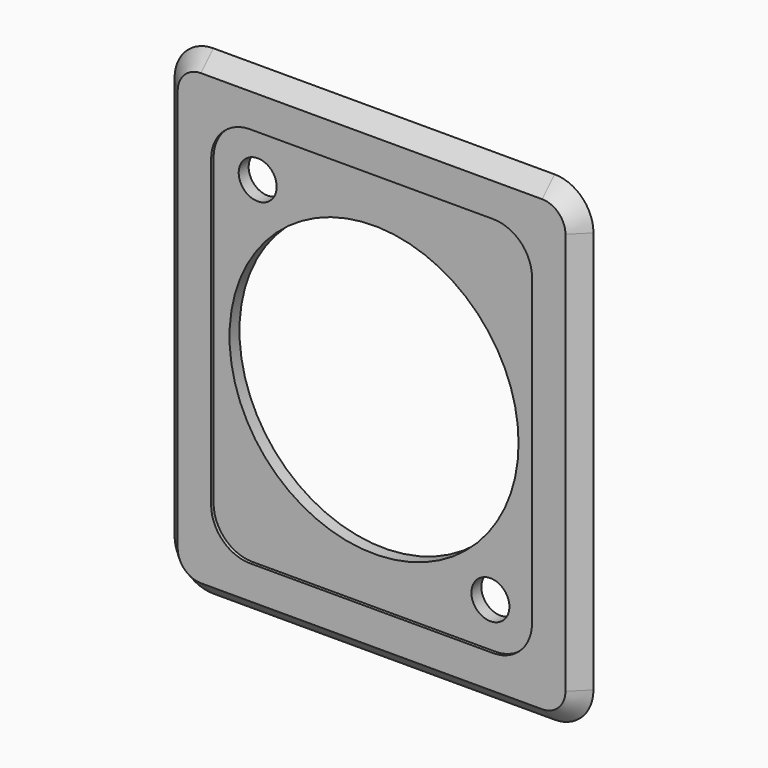
from build123d import *

# Parameters (mm, degrees)
F0_R     = 1.55
F0_R_2   = 11.8
F1_DEPTH = 1.27
F3_DEPTH = 0.254
F4_SIZE  = 1.26999


# Not quite as in the source:
# - a fillet or chamfer is up to 0.001 mm smaller than in the source, because OpenCascade refuses the exact size


with BuildPart() as f1:
    # F0 (on Front) → F1 (new body)
    with BuildSketch(Plane.XZ):
        with BuildLine():
            ThreePointArc((0, 3.175), (0.9299359697, 0.9299359697), (3.175, 0))
            Line((3.175, 0), (31.025, 0))
            ThreePointArc((31.025, 0), (33.2700640303, 0.9299359697), (34.2, 3.175))
            Line((34.2, 3.175), (34.2, 36.025))
            ThreePointArc((34.2, 36.025), (33.2700640303, 38.2700640303), (31.025, 39.2))
            Line((31.025, 39.2), (3.175, 39.2))
            ThreePointArc((3.175, 39.2), (0.9299359697, 38.2700640303), (0, 36.025))
            Line((0, 36.025), (0, 3.175))
        make_face()
        with Locations((26.5996, 7.5985)):
            Circle(F0_R, mode=Mode.SUBTRACT)
        with Locations((7.6004, 31.6015)):
            Circle(F0_R, mode=Mode.SUBTRACT)
        with Locations((17.1, 19.6)):
            Circle(F0_R_2, mode=Mode.SUBTRACT)
    extrude(amount=F1_DEPTH)

    # F2 (on face) → F3 (cut)
    with BuildSketch(Plane.XZ.offset(1.27)):
        with BuildLine():
            Line((27.025, 35.2), (7.175, 35.2))
            ThreePointArc((7.175, 35.2), (4.9299359697, 34.2700640303), (4, 32.025))
            Line((4, 32.025), (4, 7.175))
            ThreePointArc((4, 7.175), (4.9299359697, 4.9299359697), (7.175, 4))
            Line((7.175, 4), (27.025, 4))
            ThreePointArc((27.025, 4), (29.2700640303, 4.9299359697), (30.2, 7.175))
            Line((30.2, 7.175), (30.2, 32.025))
            ThreePointArc((30.2, 32.025), (29.2700640303, 34.2700640303), (27.025, 35.2))
        make_face()
    extrude(amount=-F3_DEPTH, mode=Mode.SUBTRACT)

    # F4 (size 1.27 in the source; OpenCascade refuses exactly that, so slightly less here)
    f4_edges = [f1.edges().sort_by_distance(p)[0] for p in [
        (34.2, -1.27, 19.6),
    ]]
    chamfer(f4_edges, length=F4_SIZE)


solid = f1.part
